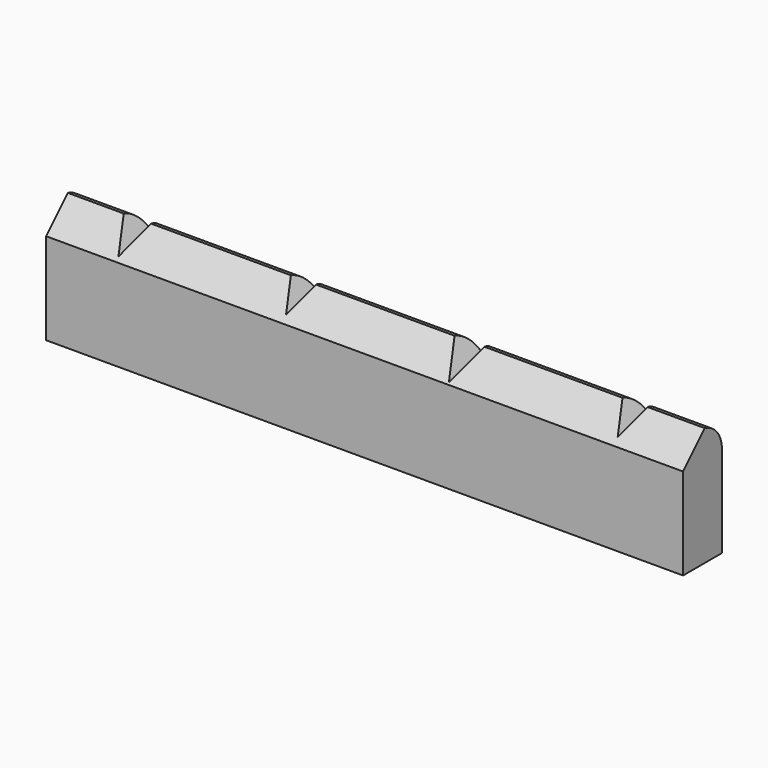
from build123d import *

# Parameters (mm, degrees)
F0_W        = 40.64
F0_H        = 3.0988
F1_DEPTH    = 7.62
F3_R        = 1.778
F4_T1_DEPTH = 49.7849047052
F5_DEPTH    = 25.4


# Not quite as in the source:
# - a fillet or chamfer that OpenCascade refuses, or shapes differently, is made with other operations: its cross-section is extruded or revolved along the edge and cut away or added


with BuildPart() as f1:
    # F0 (on Top) → F1 (new body)
    with BuildSketch(Plane.XY):
        with Locations((0, 1.5494)):
            Rectangle(F0_W, F0_H)
    extrude(amount=F1_DEPTH)

    # F3
    f3_edges = [f1.edges().sort_by_distance(p)[0] for p in [
        (0, 3.0988, 7.62),
    ]]
    fillet(f3_edges, radius=F3_R)

    # F4: chamfer of 1.778 on 1 edges, made by hand

    # F4_s2 → F4_t1 (cut)
    with BuildSketch(Plane.YZ.offset(-24.8924523526)):
        Polygon((1.778, 7.62), (0, 5.842), (0, 7.62), align=None)
    extrude(amount=F4_T1_DEPTH, mode=Mode.SUBTRACT)

    # F2 (on face) → F5 (cut)
    with BuildSketch(Plane.XZ):
        Polygon((-15.875, 6.0552954744), (-14.9716174209, 7.62), (-16.7783825791, 7.62), align=None)
        Polygon((-4.4531409051, 7.62), (-6.1132590949, 7.62), (-5.2832, 6.1822954744), align=None)
        Polygon((6.2853060633, 7.62), (4.3318939367, 7.62), (5.3086, 5.9282954744), align=None)
        Polygon((16.7050590949, 7.62), (15.0449409051, 7.62), (15.875, 6.1822954744), align=None)
    extrude(amount=-F5_DEPTH, mode=Mode.SUBTRACT)


solid = f1.part
